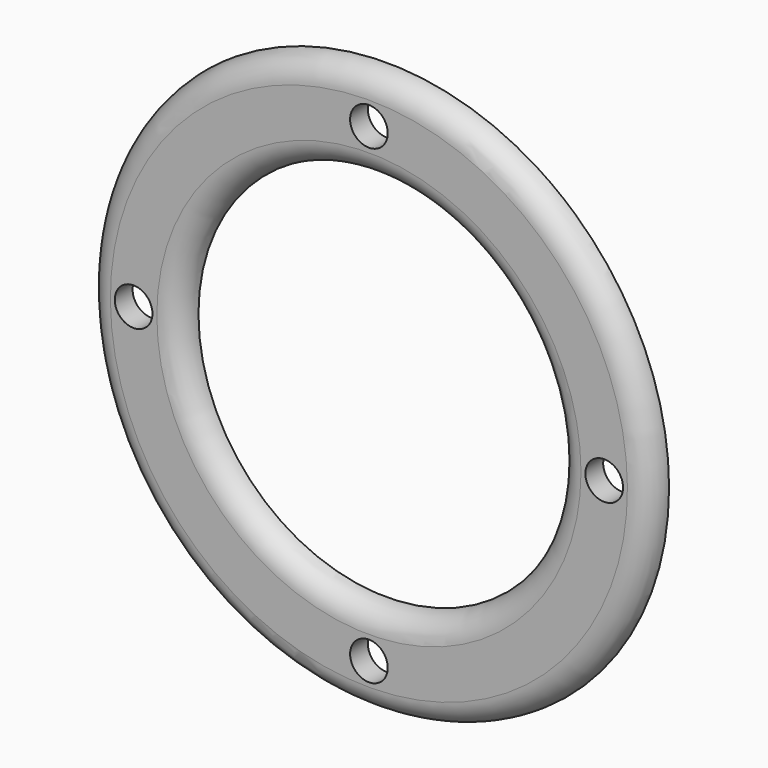
from build123d import *

# Parameters (mm, degrees)
F0_R     = 2
F1_DEPTH = 2.3622


# Not quite as in the source:
# - a fillet or chamfer that OpenCascade refuses, or shapes differently, is made with other operations: its cross-section is extruded or revolved along the edge and cut away or added


with BuildPart() as f1:
    # F0 (on Front) → F1 (new body)
    with BuildSketch(Plane.XZ):
        with BuildLine():
            Line((20, 22.360679775), (20, 0))
            ThreePointArc((20, 0), (0, -20), (-20, 0))
            Line((-20, 0), (-20, 22.360679775))
            ThreePointArc((-20, 22.360679775), (-12.2474487139, -27.3861278753), (30, 0))
            ThreePointArc((30, 0), (27.3861278753, 12.2474487139), (20, 22.360679775))
        make_face()
        with Locations((0, -25)):
            Circle(F0_R, mode=Mode.SUBTRACT)
        with Locations((-25, 0)):
            Circle(F0_R, mode=Mode.SUBTRACT)
        with Locations((25, 0)):
            Circle(F0_R, mode=Mode.SUBTRACT)
        with BuildLine():
            ThreePointArc((-16, 12), (0, 20), (16, 12))
            Line((16, 12), (16, 25.3771550809))
            ThreePointArc((16, 25.3771550809), (0, 30), (-16, 25.3771550809))
            Line((-16, 25.3771550809), (-16, 12))
        make_face()
        with Locations((0, 25)):
            Circle(F0_R, mode=Mode.SUBTRACT)
        with BuildLine():
            Line((16, 25.3771550809), (16, 12))
            ThreePointArc((16, 12), (18.973665961, 6.3245553203), (20, 0))
            Line((20, 0), (20, 22.360679775))
            ThreePointArc((20, 22.360679775), (18.0630778335, 23.9525618501), (16, 25.3771550809))
        make_face()
        with BuildLine():
            ThreePointArc((-20, 0), (-18.973665961, 6.3245553203), (-16, 12))
            Line((-16, 12), (-16, 25.3771550809))
            ThreePointArc((-16, 25.3771550809), (-18.0630778335, 23.9525618501), (-20, 22.360679775))
            Line((-20, 22.360679775), (-20, 0))
        make_face()
    extrude(amount=F1_DEPTH)

    # F2: fillet of radius 2.54 on 2 edges, made by hand

    # F2_s1 → F2_t2 (revolve, cut)
    with BuildSketch(Plane(origin=(0, 0, 0), x_dir=(0, 1, 0), z_dir=(0.8459051694, 0, 0.5333333333))):
        with BuildLine():
            ThreePointArc((0, 30), (-1.6800498325, 29.1982797174), (-2.3622, 27.4662306419))
            Line((-2.3622, 27.4662306419), (-2.3622, 30))
            Line((-2.3622, 30), (0, 30))
        make_face()
    revolve(axis=Axis((0, -2.3622, 0), (0, -1, 0)), mode=Mode.SUBTRACT)

    # F2_s3 → F2_t4 (revolve, cut)
    with BuildSketch(Plane.XY):
        with BuildLine():
            ThreePointArc((-20, 0), (-20.8017202826, -1.6800498325), (-22.5337693581, -2.3622))
            Line((-22.5337693581, -2.3622), (-20, -2.3622))
            Line((-20, -2.3622), (-20, 0))
        make_face()
    revolve(axis=Axis((0, -2.3622, 0), (0, 1, 0)), mode=Mode.SUBTRACT)


solid = f1.part
